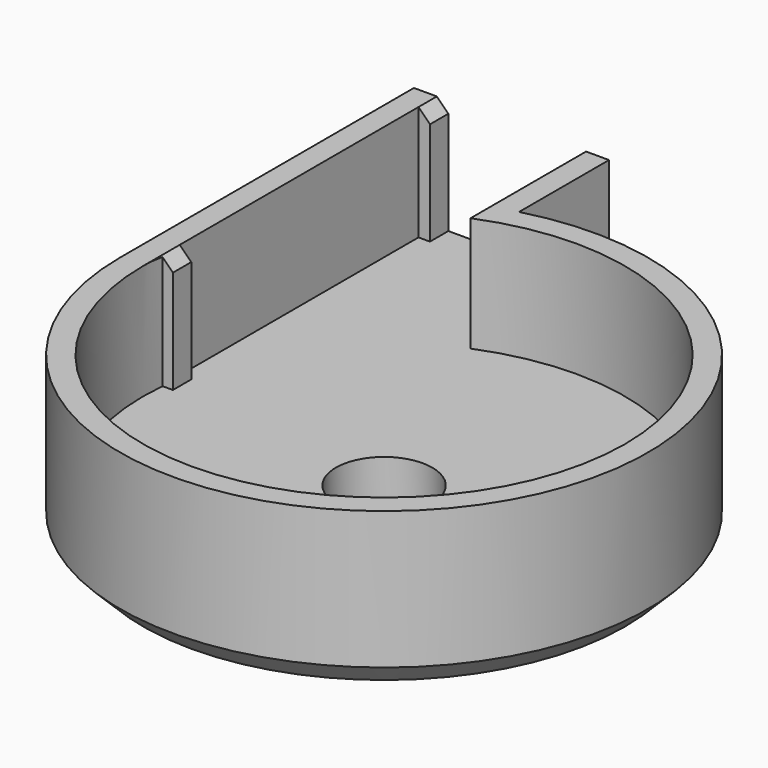
from build123d import *

# Parameters (mm, degrees)
F0_R      = 11.5
F0_R_2    = 2.1
F1_DEPTH  = 7
F2_R      = 10.5
F3_DEPTH  = 5
F5_DEPTH  = 7
F6_W      = 8.5
F6_H      = 2
F7_DEPTH  = 12.8
F8_W      = 6.5
F8_H      = 5
F9_DEPTH  = 15
F10_W     = 1
F10_H     = 5
F11_DEPTH = 0.5
F12_W     = 1
F12_H     = 5
F13_DEPTH = 0.5
F14_SIZE  = 0.49999
F15_SIZE  = 1


# Not quite as in the source:
# - a fillet or chamfer is up to 0.001 mm smaller than in the source, because OpenCascade refuses the exact size


with BuildPart() as f1:
    # F0 (on Top) → F1 (new body)
    with BuildSketch(Plane.XY):
        Circle(F0_R)
        Circle(F0_R_2, mode=Mode.SUBTRACT)
    extrude(amount=F1_DEPTH)

    # F2 (on face) → F3 (cut)
    with BuildSketch(Plane.XY.offset(7)):
        Circle(F2_R)
    extrude(amount=-F3_DEPTH, mode=Mode.SUBTRACT)

    # F4 (on face) → F5 (join)
    with BuildSketch(Plane.XY.offset(7)):
        with BuildLine():
            Line((-11.5, 16), (-11.5, 0))
            ThreePointArc((-11.5, 0), (-11.2472218792, 2.3979157617), (-10.5, 4.6904157598))
            Line((-10.5, 4.6904157598), (-10.5, 16))
            Line((-10.5, 16), (-11.5, 16))
        make_face()
        with BuildLine():
            ThreePointArc((-4, 10.7819293264), (-3.5036523196, 10.9532835453), (-3, 11.1018016556))
            Line((-3, 11.1018016556), (-3, 16))
            Line((-3, 16), (-4, 16))
            Line((-4, 16), (-4, 10.7819293264))
        make_face()
    extrude(amount=-F5_DEPTH)

    # F6 (on face) → F7 (join)
    with BuildSketch(Plane(origin=(0, 16, 0), x_dir=(-1, 0, 0), z_dir=(0, 1, 0))):
        with Locations((7.25, 1)):
            Rectangle(F6_W, F6_H)
    extrude(amount=-F7_DEPTH)

    # F8 (on face) → F9 (cut)
    with BuildSketch(Plane(origin=(0, 16, 0), x_dir=(-1, 0, 0), z_dir=(0, 1, 0))):
        with Locations((7.25, 4.5)):
            Rectangle(F8_W, F8_H)
    extrude(amount=-F9_DEPTH, mode=Mode.SUBTRACT)

    # F10 (on face) → F11 (join)
    with BuildSketch(Plane.YZ.offset(-10.5)):
        with Locations((1.5, 4.5)):
            Rectangle(F10_W, F10_H)
        with Locations((15.5, 4.5)):
            Rectangle(F10_W, F10_H)
    extrude(amount=F11_DEPTH)

    # F12 (on face) → F13 (join)
    with BuildSketch(Plane(origin=(-4, 0, 0), x_dir=(0, -1, 0), z_dir=(-1, 0, 0))):
        with Locations((-15.5, 4.5)):
            Rectangle(F12_W, F12_H)
    extrude(amount=F13_DEPTH)

    # F14 (size 0.5 in the source; OpenCascade refuses exactly that, so slightly less here)
    f14_edges = [f1.edges().sort_by_distance(p)[0] for p in [
        (-10, 1.5, 7),
        (-10, 15.5, 7),
        (-4.5, 15.5, 7),
    ]]
    chamfer(f14_edges, length=F14_SIZE)

    # F15
    f15_edges = [f1.edges().sort_by_distance(p)[0] for p in [
        (9.130991, -6.991066, 0),
        (-3, 13.550901, 0),
        (-11.5, 8, 0),
    ]]
    chamfer(f15_edges, length=F15_SIZE)


solid = f1.part
